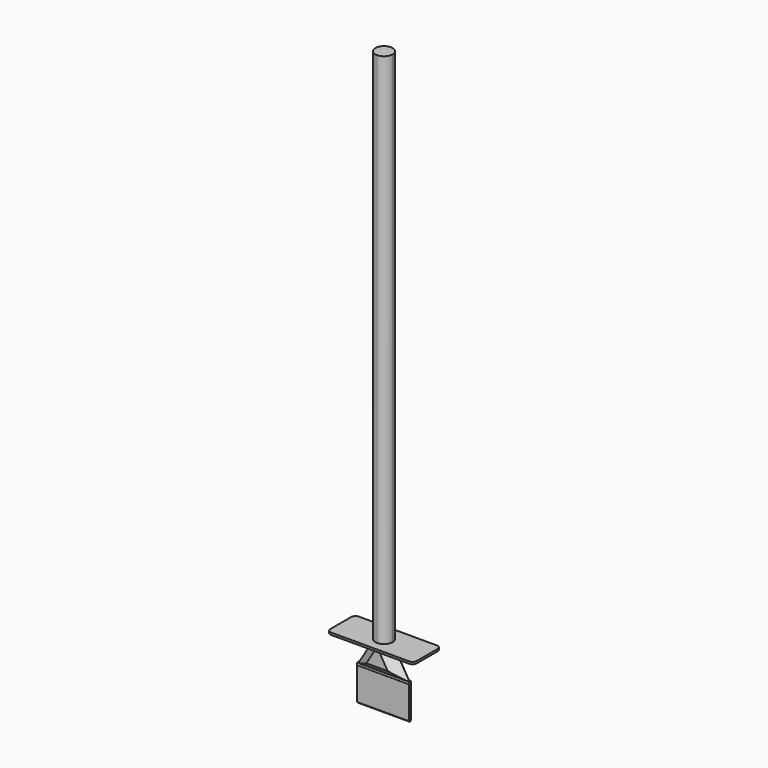
from build123d import *

# Parameters (mm, degrees)
F0_W       = 50.8
F0_H       = 1520.825
F1_DEPTH   = 25.4
F2_R       = 25.39999
F0_W_2     = 152.4
F0_H_2     = 101.6
F3_DEPTH   = 3.175
F4_DEPTH   = 25.4
F5_C1_SIZE = 25.4
F5_C2_SIZE = 25.3999
F5_C3_SIZE = 25.4
F5_C4_SIZE = 25.3999
F5_C5_SIZE = 25.4
F5_C6_SIZE = 25.3999
F6_SIZE    = 3.17499
F0_H_3     = 3.175
F7_DEPTH   = 50.8
F8_R       = 12.7
F9_SIZE    = 3.17499
F9_FACE_W  = 152.4
F9_FACE_H  = 4.4901139184


# Not quite as in the source:
# - a fillet or chamfer is up to 0.001 mm smaller than in the source, because OpenCascade refuses the exact size


with BuildPart() as f1:
    # F0 (on Front) → F1 (new body, symmetric)
    with BuildSketch(Plane.XZ):
        with Locations((0, 1.5875)):
            Rectangle(F0_W, F0_H)
    extrude(amount=F1_DEPTH, both=True)

    # F2 (radius 25.4 in the source; OpenCascade refuses exactly that, so slightly less here)
    f2_edges = [f1.edges().sort_by_distance(p)[0] for p in [
        (-25.4, -25.4, 1.5875),
        (25.4, -25.4, 1.5875),
        (25.4, 25.4, 1.5875),
        (-25.4, 25.4, 1.5875),
    ]]
    fillet(f2_edges, radius=F2_R)


with BuildPart() as f3:
    # F0 (on Front) → F3 (new body, symmetric)
    with BuildSketch(Plane.XZ):
        with Locations((0, -897.9075126523)):
            Rectangle(F0_W_2, F0_H_2)
    extrude(amount=F3_DEPTH, both=True)

    # F6 (size 3.175 in the source; OpenCascade refuses exactly that, so slightly less here)
    f6_edges = [f3.edges().sort_by_distance(p)[0] for p in [
        (0, 3.175, -948.707513),
        (0, -3.175, -948.707513),
    ]]
    chamfer(f6_edges, length=F6_SIZE)

    # F9 (size 3.175 in the source; OpenCascade refuses exactly that, so slightly less here)
    f9_edges = [f3.edges().sort_by_distance(p)[0] for p in [
        (0, 3.175, -847.107513),
        (0, -3.175, -847.107513),
    ]]
    chamfer(f9_edges, length=F9_SIZE)


with BuildPart() as f4:
    # F0 (on Front) → F4 (new body, symmetric)
    with BuildSketch(Plane.XZ):
        Polygon((27.2951323446, -765.175), (-27.2951323446, -765.175), (-76.2, -847.1075126523), (76.2, -847.1075126523), align=None)
    extrude(amount=F4_DEPTH, both=True)

    # F5: chamfer of 25.4 on 6 edges, made by hand

    # F5_c1
    f5_c1_edges = [f4.edges().sort_by_distance(p)[0] for p in [
        (51.7475661723, 25.4, -806.1412563261),
    ]]
    chamfer(f5_c1_edges, length=F5_C1_SIZE)

    # F5_c2 (size 25.4 in the source; OpenCascade refuses exactly that, so slightly less here)
    f5_c2_edges = [f4.edges().sort_by_distance(p)[0] for p in [
        (51.7475661723, -25.4, -806.1412563261),
    ]]
    chamfer(f5_c2_edges, length=F5_C2_SIZE)

    # F5_c3
    f5_c3_edges = [f4.edges().sort_by_distance(p)[0] for p in [
        (-14.7903490716, 25.4, -847.1075126523),
    ]]
    chamfer(f5_c3_edges, length=F5_C3_SIZE)

    # F5_c4 (size 25.4 in the source; OpenCascade refuses exactly that, so slightly less here)
    f5_c4_edges = [f4.edges().sort_by_distance(p)[0] for p in [
        (-14.7902908419, -25.4, -847.1075126523),
    ]]
    chamfer(f5_c4_edges, length=F5_C4_SIZE)

    # F5_c5
    f5_c5_edges = [f4.edges().sort_by_distance(p)[0] for p in [
        (-44.1670367937, 25.4, -793.4412563261),
    ]]
    chamfer(f5_c5_edges, length=F5_C5_SIZE)

    # F5_c6 (size 25.4 in the source; OpenCascade refuses exactly that, so slightly less here)
    f5_c6_edges = [f4.edges().sort_by_distance(p)[0] for p in [
        (-44.1670666383, -25.4, -793.4413063261),
    ]]
    chamfer(f5_c6_edges, length=F5_C6_SIZE)


with BuildPart() as f7:
    # F0 (on Front) → F7 (new body, symmetric)
    with BuildSketch(Plane.XZ):
        Polygon((127, -758.825), (25.4, -758.825), (25.4, -762), (27.2951323446, -765.175), (127, -765.175), align=None)
        Polygon((-25.4, -762), (-25.4, -758.825), (-127, -758.825), (-127, -765.175), (-27.2951323446, -765.175), align=None)
        with Locations((0, -760.4125)):
            Rectangle(F0_W, F0_H_3)
        Polygon((25.4, -762), (-25.4, -762), (-27.2951323446, -765.175), (27.2951323446, -765.175), align=None)
    extrude(amount=F7_DEPTH, both=True)

    # F8
    f8_edges = [f7.edges().sort_by_distance(p)[0] for p in [
        (127, 50.8, -762),
        (127, -50.8, -762),
        (-127, -50.8, -762),
        (-127, 50.8, -762),
    ]]
    fillet(f8_edges, radius=F8_R)


with BuildPart() as f10:
    # F9_face (on face) → F10 (revolve)
    with BuildSketch(Plane(origin=(0, -1.587505, -848.6950076523), x_dir=(1, 0, 0), z_dir=(0, -0.7071067812, 0.7071067812))):
        Rectangle(F9_FACE_W, F9_FACE_H)
    revolve(axis=Axis((0, 0, -847.1075126523), (-1, 0, 0)))


solid = Compound([f1.part, f3.part, f4.part, f7.part, f10.part])
